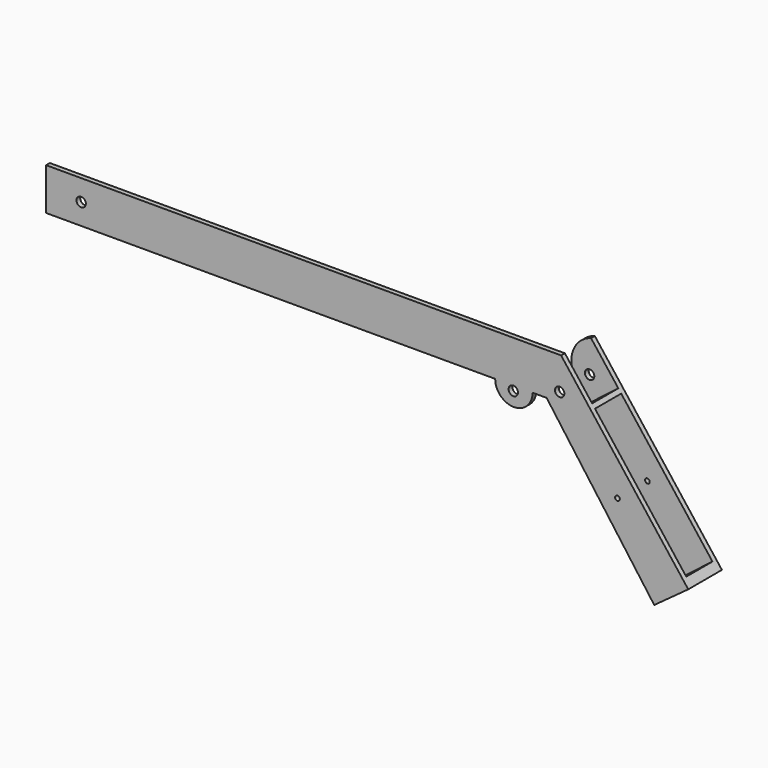
from build123d import *

# Parameters (mm, degrees)
F1_DEPTH  = 9
F3_DEPTH  = 8
F4_W      = 7
F4_H      = 42.4595763843
F4_H_2    = 6.157477504
F5_DEPTH  = 111.888617615
F7_DEPTH  = 9
F8_R      = 1
F8_R_2    = 0.5
F9_DEPTH  = 9.001
F10_R     = 1
F11_DEPTH = 9.001


# Not quite as in the source:
# - a feature names something its author has since deleted; it is built from what else it names


with BuildPart() as f1:
    # F0 (on Front) → F1 (new body)
    with BuildSketch(Plane.XZ):
        Polygon((-64.9861803949, 9), (-64.9861803949, 0), (31.0138196051, 0), (39.0138196051, 0), (42.0138196051, 0), (65.0138196051, -31.496031496), (72.2821345657, -26.1883391884), (45.1079792442, 9), align=None)
        with BuildLine():
            Line((39.0138196051, 0), (31.0138196051, 0))
            ThreePointArc((31.0138196051, 0), (35.0138196051, -4), (39.0138196051, 0))
        make_face()
    extrude(amount=F1_DEPTH)

    # F2 (on face) → F3 (cut)
    with BuildSketch(Plane(origin=(0, 0, 0), x_dir=(-1, 0, 0), z_dir=(0, 1, 0))):
        with BuildLine():
            ThreePointArc((-45.1079792442, 9), (-41.2127769921, 5.307273962), (-42.0138196051, 0))
            Line((-42.0138196051, 0), (-39.0138196051, 0))
            ThreePointArc((-39.0138196051, 0), (-35.0138196051, -4), (-31.0138196051, 0))
            Line((-31.0138196051, 0), (64.9861803949, 0))
            Line((64.9861803949, 0), (64.9861803949, 9))
            Line((64.9861803949, 9), (-45.1079792442, 9))
        make_face()
    extrude(amount=-F3_DEPTH, mode=Mode.SUBTRACT)

    # F4 (on face) → F5 (cut, through all)
    with BuildSketch(Plane(origin=(32.6104059702, 0, 25.1833492962), x_dir=(0, 1, 0), z_dir=(0.7914681616, 0, 0.6112103968))):
        with Locations((-4.5, -41.6770406282)):
            Rectangle(F4_W, F4_H)
        with Locations((-4.5, -17.368513684)):
            Rectangle(F4_W, F4_H_2)
    extrude(amount=-F5_DEPTH, mode=Mode.SUBTRACT)

    # F6 (on face) → F7 (join)
    with BuildSketch(Plane.XZ.offset(9)):
        Polygon((45.0138196051, -4.1081780212), (51.5466572041, 0.662431406), (50.9354468073, 1.4538995677), (44.551974041, -3.4757300893), align=None)
    extrude(amount=-F7_DEPTH)

    # F8 (on face) → F9 (cut, through all)
    with BuildSketch(Plane.XZ.offset(9)):
        with Locations((44.8008679783, 2.0352441098)):
            Circle(F8_R)
        with Locations((57.1549696039, -13.9623209745)):
            Circle(F8_R_2)
        with Locations((-57.4861803949, 4.5)):
            Circle(F8_R)
    extrude(amount=-F9_DEPTH, mode=Mode.SUBTRACT)

    # F10 (on face) → F11 (cut, through all)
    with BuildSketch(Plane.XZ.offset(9)):
        with Locations((-60.9861803949, -1.4662119793)):
            Circle(F10_R)
        with Locations((34.8888196051, -0.9921567416)):
            Circle(F10_R)
    extrude(amount=-F11_DEPTH, mode=Mode.SUBTRACT)


solid = f1.part
